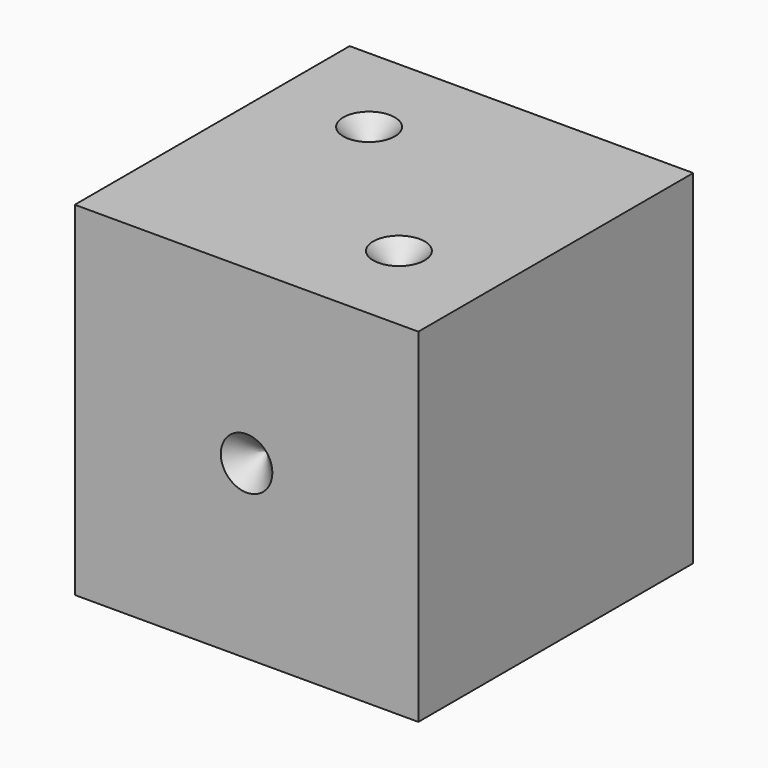
from build123d import *

# Parameters (mm, degrees)
F0_W     = 20
F0_H     = 20
F1_DEPTH = 20
F2_R     = 1.5
F3_DEPTH = 1.5
F4_R     = 1.5
F5_DEPTH = 1.5
F6_SIZE  = 1.49999


# Not quite as in the source:
# - a fillet or chamfer is up to 0.001 mm smaller than in the source, because OpenCascade refuses the exact size


with BuildPart() as f1:
    # F0 (on Top) → F1 (new body)
    with BuildSketch(Plane.XY):
        with Locations((10, 10)):
            Rectangle(F0_W, F0_H)
    extrude(amount=F1_DEPTH)

    # F2 (on face) → F3 (cut)
    with BuildSketch(Plane.XZ):
        with Locations((10, 10)):
            Circle(F2_R)
    extrude(amount=-F3_DEPTH, mode=Mode.SUBTRACT)

    # F4 (on face) → F5 (cut)
    with BuildSketch(Plane.XY.offset(20)):
        with Locations((5.6568542495, 14.3431457505)):
            Circle(F4_R)
        with Locations((14.3431457505, 5.6568542495)):
            Circle(F4_R)
    extrude(amount=-F5_DEPTH, mode=Mode.SUBTRACT)

    # F6 (size 1.5 in the source; OpenCascade refuses exactly that, so slightly less here)
    f6_edges = [f1.edges().sort_by_distance(p)[0] for p in [
        (8.5, 1.5, 10),
        (4.156854, 14.343146, 18.5),
        (12.843146, 5.656854, 18.5),
    ]]
    chamfer(f6_edges, length=F6_SIZE)


solid = f1.part
